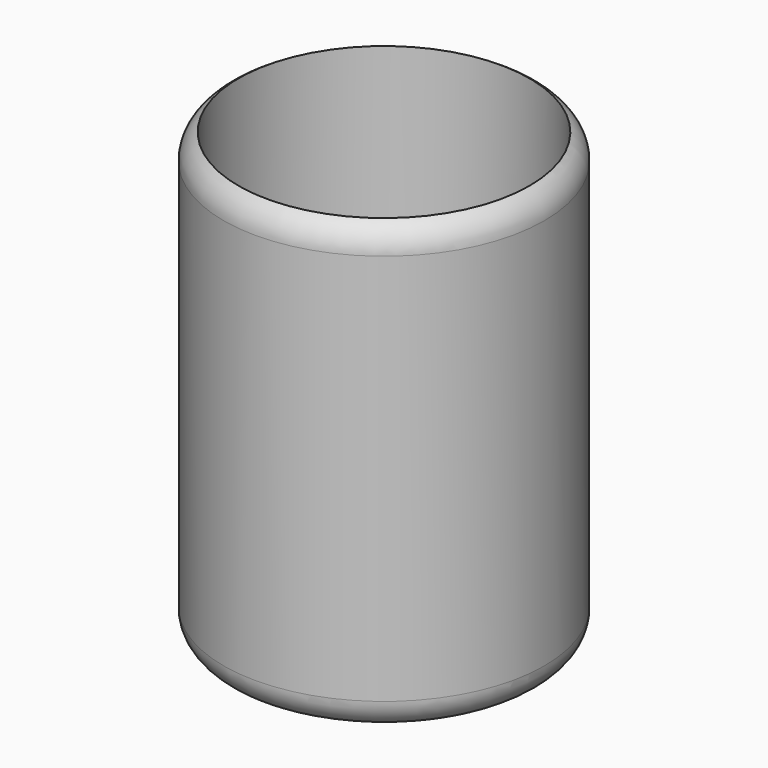
from build123d import *

# Parameters (mm, degrees)
F0_R     = 26.884522514
F1_DEPTH = 75
F2_T     = -2.5
F4_R     = 5


# Not quite as in the source:
# - a fillet or chamfer that OpenCascade refuses, or shapes differently, is made with other operations: its cross-section is extruded or revolved along the edge and cut away or added


with BuildPart() as f1:
    # F0 (on Top) → F1 (new body)
    with BuildSketch(Plane.XY):
        Circle(F0_R)
    extrude(amount=F1_DEPTH)

    # F2
    f2_openings = [f1.faces().sort_by_distance(p)[0] for p in [
        (0, 0, 75),
    ]]
    offset(amount=F2_T, openings=f2_openings)

    # F3: fillet of radius 5 on 1 edges, made by hand

    # F3_s1 → F3_t2 (revolve, cut)
    with BuildSketch(Plane.XZ):
        with BuildLine():
            ThreePointArc((26.884522514, 70.6698729811), (26.2146495329, 73.1698729811), (24.384522514, 75))
            Line((24.384522514, 75), (26.884522514, 75))
            Line((26.884522514, 75), (26.884522514, 70.6698729811))
        make_face()
    revolve(axis=Axis((0, 0, 75), (0, 0, 1)), mode=Mode.SUBTRACT)

    # F4
    f4_edges = [f1.edges().sort_by_distance(p)[0] for p in [
        (-26.884523, 0, 0),
    ]]
    fillet(f4_edges, radius=F4_R)


solid = f1.part
